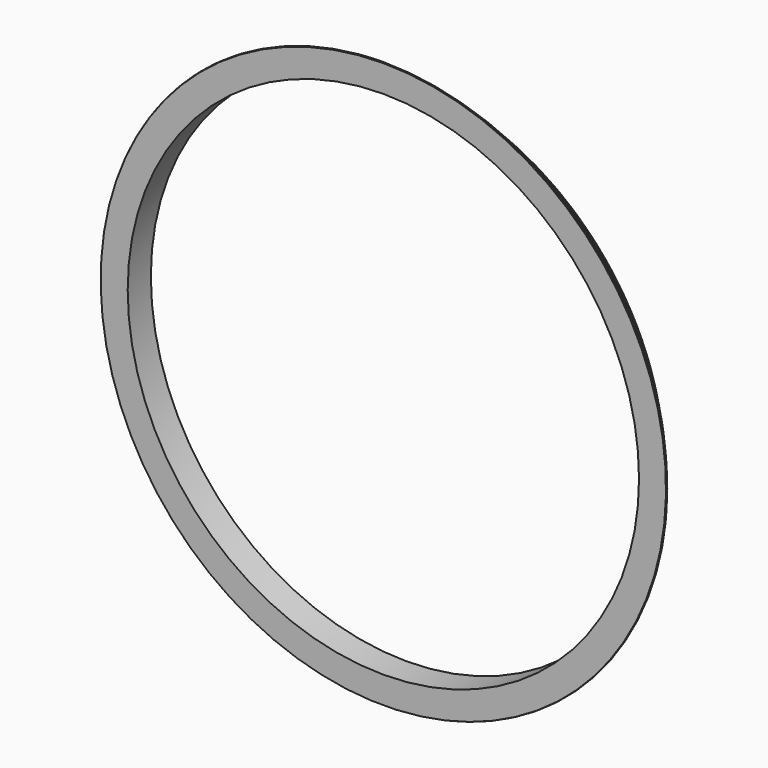
from build123d import *


with BuildPart() as f1:
    # F0 (on Right) → F1 (revolve)
    with BuildSketch(Plane.YZ):
        with BuildLine():
            Line((0, 93.0275), (0, 84.1375))
            Line((0, 84.1375), (9.525, 84.1375))
            add(Edge.make_bspline(
                [(0, 93.0275), (0.2088990535, 93.081663291), (0.6861026497, 93.2053925124), (0.3759666943, 92.1426495892), (0.8114380473, 91.6420579009), (2.484088711, 91.5563355103), (3.2963665543, 90.4876015981), (3.216440736, 89.0719694166), (5.3714175986, 89.6248800904), (5.9465206782, 85.3425098548), (8.83795984, 86.566069281), (7.6335785616, 84.3012759174), (9.6128037423, 85.0953242376), (9.5513664398, 84.4251234478), (9.525, 84.1375)],
                knots=[0, 0, 0, 0, 0.0539660272, 0.1232785972, 0.1809072688, 0.2768820626, 0.3633316286, 0.4410411497, 0.5325609458, 0.6725491168, 0.7712576154, 0.8540158261, 0.9373494152, 1, 1, 1, 1], degree=3))
        make_face()
    revolve(axis=Axis((0, 0.8836919442, 0), (0, 1, 0)))


solid = f1.part
